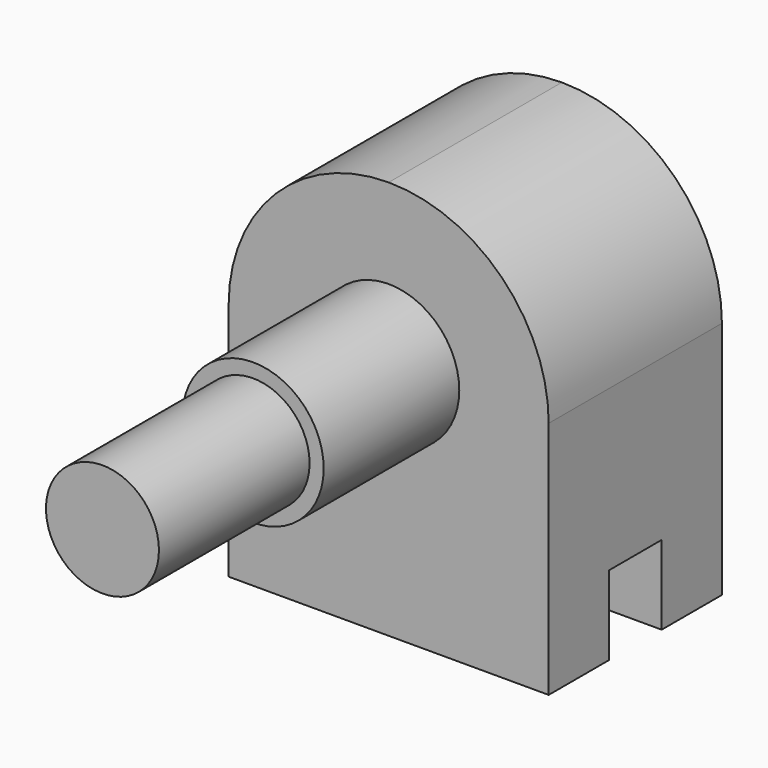
from build123d import *

# Parameters (mm, degrees)
F0_W     = 17
F0_H     = 17
F1_DEPTH = 11.5
F2_R     = 3.75
F3_DEPTH = 9
F4_R     = 3
F5_DEPTH = 10
F6_W     = 17
F6_H     = 4
F7_DEPTH = 4.2
F8_R     = 8.49999


# Not quite as in the source:
# - a fillet or chamfer is up to 0.001 mm smaller than in the source, because OpenCascade refuses the exact size


with BuildPart() as f1:
    # F0 (on Front) → F1 (new body)
    with BuildSketch(Plane.XZ):
        Rectangle(F0_W, F0_H)
    extrude(amount=F1_DEPTH)

    # F2 (on face) → F3 (join)
    with BuildSketch(Plane.XZ.offset(11.5)):
        Circle(F2_R)
    extrude(amount=F3_DEPTH)

    # F4 (on face) → F5 (join)
    with BuildSketch(Plane.XZ.offset(20.5)):
        Circle(F4_R)
    extrude(amount=F5_DEPTH)

    # F6 (on face) → F7 (join)
    with BuildSketch(Plane(origin=(0, 0, -8.5), x_dir=(1, 0, 0), z_dir=(0, 0, -1))):
        with Locations((0, 2)):
            Rectangle(F6_W, F6_H)
        with Locations((0, 9.5)):
            Rectangle(F6_W, F6_H)
    extrude(amount=F7_DEPTH)

    # F8 (radius 8.5 in the source; OpenCascade refuses exactly that, so slightly less here)
    f8_edges = [f1.edges().sort_by_distance(p)[0] for p in [
        (8.5, -5.75, 8.5),
        (-8.5, -5.75, 8.5),
    ]]
    fillet(f8_edges, radius=F8_R)


solid = f1.part
